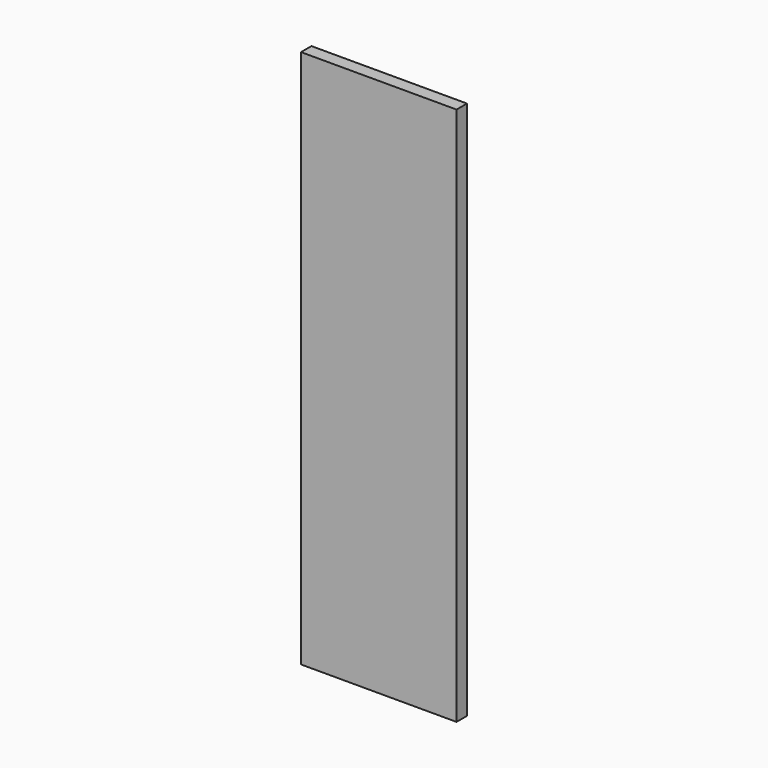
from build123d import *

# Parameters (mm, degrees)
F1_DEPTH = 1.6


# Not quite as in the source:
# - a feature names something its author has since deleted; it is built from what else it names


with BuildPart() as f1:
    # F0 (on Front) → F1 (new body)
    with BuildSketch(Plane.XZ):
        Polygon((8.975, 66.04), (8.975, 0), (18.5, 0), (28.025, 0), (28.025, 66.04), align=None)
    extrude(amount=F1_DEPTH)


solid = f1.part
